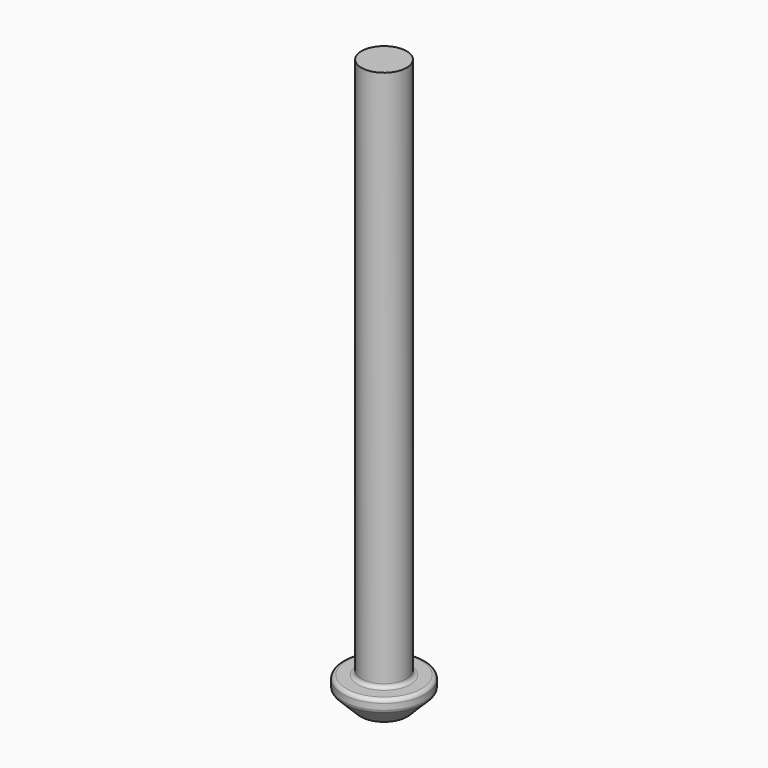
from build123d import *

# Parameters (mm, degrees)
F1_R     = 2.75
F1_R_2   = 1.5
F2_DEPTH = 2
F3_START = 1.5
F3_DEPTH = 0.5
F4_START = 2
F4_DEPTH = 36
F5_SIZE2 = 1.25
F5_SIZE  = 1.25
F6_R     = 0.25


# Not quite as in the source:
# - a feature names something its author has since deleted; it is built from what else it names


with BuildPart() as f2:
    # F1 (on Top) → F2 (new body)
    with BuildSketch(Plane.XY):
        Circle(F1_R)
        Circle(F1_R_2, mode=Mode.SUBTRACT)
        Circle(F1_R_2)
        Polygon((-0.5773502692, -1), (-1.1547005384, 0), (-0.5773502692, 1), (0.5773502692, 1), (1.1547005384, 0), (0.5773502692, -1), align=None, mode=Mode.SUBTRACT)
    extrude(amount=F2_DEPTH)

    # F1 (on Top) → F3 (join)
    with BuildSketch(Plane.XY.offset(F3_START)):
        Polygon((-0.5773502692, 1), (-1.1547005384, 0), (-0.5773502692, -1), (0.5773502692, -1), (1.1547005384, 0), (0.5773502692, 1), align=None)
    extrude(amount=F3_DEPTH)

    # F1 (on Top) → F4 (join)
    with BuildSketch(Plane.XY.offset(F4_START)):
        Circle(F1_R_2)
        Polygon((-0.5773502692, -1), (-1.1547005384, 0), (-0.5773502692, 1), (0.5773502692, 1), (1.1547005384, 0), (0.5773502692, -1), align=None, mode=Mode.SUBTRACT)
        Polygon((-0.5773502692, 1), (-1.1547005384, 0), (-0.5773502692, -1), (0.5773502692, -1), (1.1547005384, 0), (0.5773502692, 1), align=None)
    extrude(amount=F4_DEPTH)

    # F5
    f5_edges = [f2.edges().sort_by_distance(p)[0] for p in [
        (-2.75, 0, 0),
    ]]
    chamfer(f5_edges, length=F5_SIZE, length2=F5_SIZE2)

    # F6
    f6_edges = [f2.edges().sort_by_distance(p)[0] for p in [
        (-2.75, 0, 2),
        (-1.5, 0, 2),
        (-1.5, 0, 0),
        (-2.75, 0, 1.25),
    ]]
    fillet(f6_edges, radius=F6_R)


solid = f2.part
